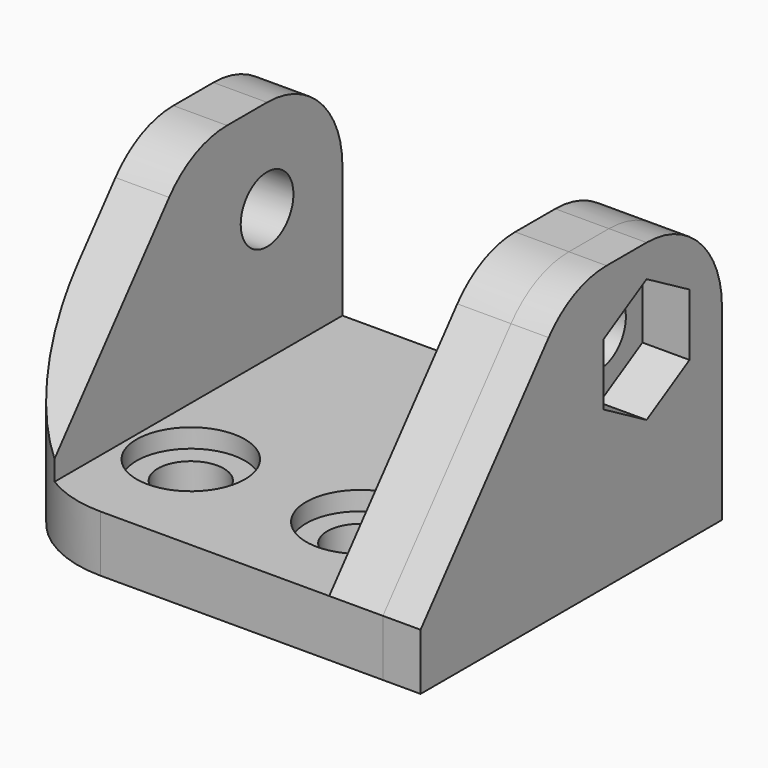
from build123d import *

# Parameters (mm, degrees)
F0_W      = 21
F0_H      = 20
F1_DEPTH  = 3
F2_W      = 2.85
F2_H      = 20
F3_DEPTH  = 12
F4_R      = 6
F5_R      = 1.75
F6_DEPTH  = 21.001
F7_R      = 5
F8_R      = 1.75
F9_DEPTH  = 3.001
F10_DEPTH = 2
F12_DEPTH = 2.5
F13_R     = 2.875
F14_DEPTH = 1


with BuildPart() as f1:
    # F0 (on Top) → F1 (new body)
    with BuildSketch(Plane.XY):
        with Locations((10.5, 10)):
            Rectangle(F0_W, F0_H)
    extrude(amount=F1_DEPTH)

    # F2 (on face) → F3 (join)
    with BuildSketch(Plane.XY.offset(3)):
        with Locations((1.425, 10)):
            Rectangle(F2_W, F2_H)
        with Locations((19.575, 10)):
            Rectangle(F2_W, F2_H)
    extrude(amount=F3_DEPTH)

    # F4
    f4_edges = [f1.edges().sort_by_distance(p)[0] for p in [
        (0, 0, 7.5),
    ]]
    fillet(f4_edges, radius=F4_R)

    # F5 (on face) → F6 (cut, through all)
    with BuildSketch(Plane(origin=(0, 0, 0), x_dir=(0, -1, 0), z_dir=(-1, 0, 0))):
        with Locations((-15, 10)):
            Circle(F5_R)
        Polygon((0, 15), (-10, 15), (0, 3), align=None)
    extrude(amount=-F6_DEPTH, mode=Mode.SUBTRACT)

    # F7
    f7_edges = [f1.edges().sort_by_distance(p)[0] for p in [
        (1.425, 20, 15),
        (19.575, 20, 15),
        (1.425, 10, 15),
        (19.575, 10, 15),
    ]]
    fillet(f7_edges, radius=F7_R)

    # F8 (on face) → F9 (cut, through all)
    with BuildSketch(Plane.XY.offset(3)):
        with Locations((6, 6)):
            Circle(F8_R)
        with Locations((15, 6)):
            Circle(F8_R)
    extrude(amount=-F9_DEPTH, mode=Mode.SUBTRACT)

    # F10 (add): a face of the model
    f10_faces = [f1.faces().sort_by_distance(p)[0] for p in [
        (21, 11.3560605972, 6.2794868265),
    ]]
    extrude(f10_faces, amount=F10_DEPTH)

    # F11 (on face) → F12 (cut)
    with BuildSketch(Plane.YZ.offset(23)):
        Polygon((17.85, 8.3545517328), (17.85, 11.6454482672), (15, 13.2908965344), (12.15, 11.6454482672), (12.15, 8.3545517328), (15, 6.7091034656), align=None)
    extrude(amount=-F12_DEPTH, mode=Mode.SUBTRACT)

    # F13 (on face) → F14 (cut)
    with BuildSketch(Plane.XY.offset(3)):
        with Locations((6, 6)):
            Circle(F13_R)
        with Locations((15, 6)):
            Circle(F13_R)
    extrude(amount=-F14_DEPTH, mode=Mode.SUBTRACT)


solid = f1.part
